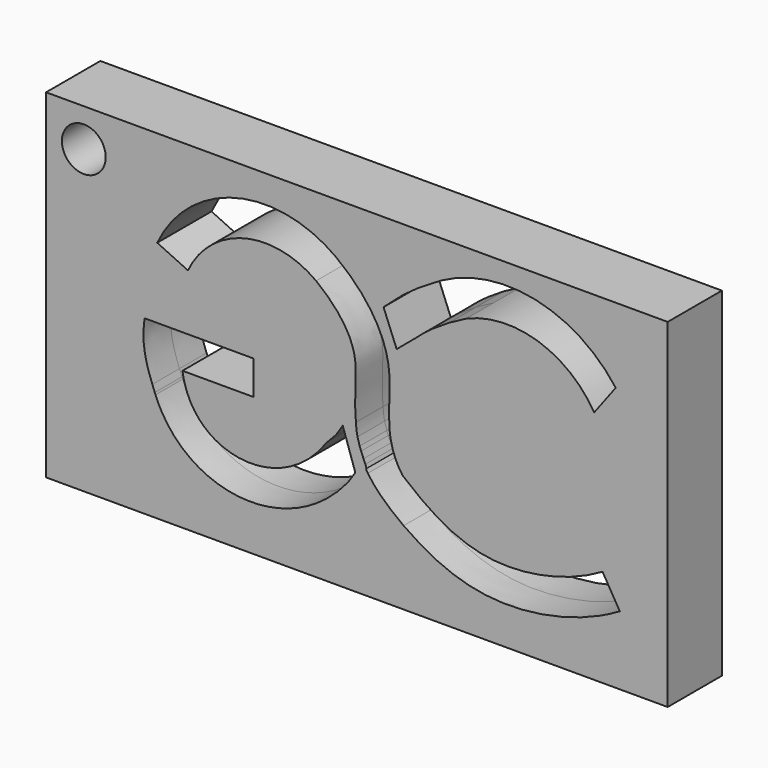
from build123d import *

# Parameters (mm, degrees)
F0_W     = 55
F0_H     = 30
F0_R     = 1.9388659874
F1_DEPTH = 3


# Not quite as in the source:
# - ends of sketch curves that miss each other by under 0.0002 mm in the source are joined
# - the dataset's text gives a spline's control points without its knots; the knots are read off the source's solid


with BuildPart() as f1:
    # F0 (on Front) → F1 (new body, symmetric)
    with BuildSketch(Plane.XZ):
        Rectangle(F0_W, F0_H)
        with Locations((-24.1624657065, 11.6540621966)):
            Circle(F0_R, mode=Mode.SUBTRACT)
        with BuildLine():
            ThreePointArc((-17.6640928467, 6.4768509395), (-10.685556205, 12.2426405249), (-1.8066326116, 10.4793994675))
            add(Edge.make_bspline(
                [(-1.8066326116, 10.4793994675), (0.9111458785, 8.4068691358), (4.1202484659, 3.5315186205), (2.1705021087, -1.9989735062), (4.045421263, -4.5930928496)],
                knots=[0, 0, 0, 0, 0.5094502434, 1, 1, 1, 1], degree=3))
            add(Edge.make_bspline(
                [(4.045421263, -4.5930928496), (6.4784704527, -6.6385440032), (11.4225557915, -9.8002947462), (18.8378328842, -8.054314346), (21.7365036724, -6.3367947143)],
                knots=[0, 0, 0, 0, 0.4804113206, 1, 1, 1, 1], degree=3))
            Line((21.7365036724, -6.3367947143), (23.2657495656, -8.9177648804))
            add(Edge.make_bspline(
                [(4.1382202245, -8.4692971196), (4.1624678344, -8.4865837301), (4.9099788848, -9.0175085674), (6.0687236287, -9.7483352983), (7.7170833942, -10.5320442339), (9.0266705688, -11.015570061), (10.1790279052, -11.3156937619), (11.1349042612, -11.4860935206), (12.1118572673, -11.6074297366), (13.3407082821, -11.6664441259), (15.3172141164, -11.5856834284), (17.7803139056, -11.1846498348), (20.641174588, -10.2819941321), (22.4229996015, -9.4171091932), (23.2657495656, -8.9177648804)],
                knots=[0.1208031529, 0.1208031529, 0.1208031529, 0.1208031529, 0.125, 0.25, 0.3125, 0.375, 0.4375, 0.46875, 0.5, 0.5625, 0.625, 0.75, 0.875, 0.9999989076, 0.9999989076, 0.9999989076, 0.9999989076], degree=3))
            add(Edge.make_bspline(
                [(0.9708350698, -5.4183705026), (1.6910337242, -6.5228260499), (2.8786849452, -7.5505327146), (4.1382202245, -8.4692971196)],
                knots=[0.5007210761, 0.5007210761, 0.5007210761, 0.5007210761, 1, 1, 1, 1], degree=3))
            add(Edge.make_bspline(
                [(0.7749087459, -5.0950080167), (0.8355835769, -5.2034973247), (0.9010125029, -5.3112945995), (0.9708350698, -5.4183705026)],
                knots=[0.4523164645, 0.4523164645, 0.4523164645, 0.4523164645, 0.5007210761, 0.5007210761, 0.5007210761, 0.5007210761], degree=3))
            add(Edge.make_bspline(
                [(0.6601995359, -4.87802362), (0.696432638, -4.9506366895), (0.7346227712, -5.0229748944), (0.7749087459, -5.0950080167)],
                knots=[0.4201774883, 0.4201774883, 0.4201774883, 0.4201774883, 0.4523164645, 0.4523164645, 0.4523164645, 0.4523164645], degree=3))
            add(Edge.make_bspline(
                [(0.6601995359, -4.87802362), (0.5457553685, -4.9921466011), (-0.197418957, -5.679000658), (-0.8276000802, -7.3815559883), (-3.5383820349, -9.5528269631), (-6.4036037178, -10.878806976), (-9.5175268759, -11.3250409398), (-12.5958587504, -10.8244366378), (-14.9118581064, -9.5196831868), (-16.4503468255, -7.9236394551), (-17.3737530763, -6.5629717915), (-17.9697890031, -5.3603946032), (-18.0825537585, -4.7711814756), (-18.0964615136, -4.6896541748)],
                knots=[0.0363625791, 0.0363625791, 0.0363625791, 0.0363625791, 0.0512646152, 0.1224303682, 0.2066568702, 0.2887928045, 0.3697104631, 0.4503939374, 0.5250439069, 0.5926719237, 0.6520324546, 0.7122837255, 0.7221646459, 0.7221646459, 0.7221646459, 0.7221646459], degree=3))
            add(Edge.make_bspline(
                [(-18.786193803, 0.233763308), (-19.1042212428, -1.8131556769), (-18.6276745861, -3.2945041185), (-18.0964615136, -4.6896541748)],
                knots=[0, 0, 0, 0, 4.8787183272, 4.8787183272, 4.8787183272, 4.8787183272], degree=3))
            Line((-18.786193803, 0.233763308), (-9.1412619867, 0.233763308))
            Line((-9.1412619867, 0.233763308), (-9.1412619867, -2.766236692))
            Line((-9.1412619867, -2.766236692), (-11.708700146, -2.766236692))
            add(Edge.make_bspline(
                [(-11.708700146, -2.766236692), (-8.4560263125, -2.815236385), (-4.719044159, -3.0335808655), (-2.1487066373, -3.3793081037)],
                knots=[0.87686085, 0.87686085, 0.87686085, 0.87686085, 0.9540771145, 0.9540771145, 0.9540771145, 0.9540771145], degree=3))
            add(Edge.make_bspline(
                [(-2.1487066373, -3.3793081037), (-2.0687729336, -3.3900597106), (-1.9899675131, -3.4009345117), (-1.9123400298, -3.4119312449)],
                knots=[0.9540771145, 0.9540771145, 0.9540771145, 0.9540771145, 0.9564784264, 0.9564784264, 0.9564784264, 0.9564784264], degree=3))
            Line((-1.9123400298, -3.4119312449), (-1.8364996879, -3.3321739989))
            Line((-1.8364996879, -3.3321739989), (-1.2497392903, -2.4288706426))
            Line((-1.2497392903, -2.4288706426), (-0.8619702149, -3.5822052172))
            add(Edge.make_bspline(
                [(-0.8619702149, -3.5822052172), (-0.4110593021, -3.6667089832), (-0.0287691917, -3.7568014187), (0.2682413254, -3.8520591098)],
                knots=[0.9682440451, 0.9682440451, 0.9682440451, 0.9682440451, 0.9849297687, 0.9849297687, 0.9849297687, 0.9849297687], degree=3))
            add(Edge.make_bspline(
                [(0.0566001038, -2.8747222202), (0.1099315572, -3.2013897212), (0.1766725727, -3.5279972379), (0.2682413254, -3.8520591098)],
                knots=[0.1312140251, 0.1312140251, 0.1312140251, 0.1312140251, 0.2709870602, 0.2709870602, 0.2709870602, 0.2709870602], degree=3))
            add(Edge.make_bspline(
                [(-0.0856948489, -1.7935240537), (-0.0651666036, -2.2040296052), (-0.0140771955, -2.5577803712), (0.0566001038, -2.8747222202)],
                knots=[0, 0, 0, 0, 0.9044663432, 0.9044663432, 0.9044663432, 0.9044663432], degree=3))
            add(Edge.make_bspline(
                [(-3.6107100667, 8.0823726543), (-3.0624362988, 7.6631509681), (-2.0964601547, 6.8016967531), (-1.2314902531, 5.7195620145), (-0.7330802188, 4.8707855584), (-0.4512938807, 4.2466244067), (-0.287727537, 3.7365048832), (-0.1965285589, 3.3315021794), (-0.1475436674, 3.0291795886), (-0.1171491383, 2.7232253787), (-0.1006872263, 2.367601974), (-0.098417222, 1.9711308495), (-0.1106132344, 1.3862202996), (-0.1452655215, 0.5543107318), (-0.1679299933, -0.5614993222), (-0.1282499701, -1.3843821047), (-0.0856948489, -1.7935240537)],
                knots=[0.0011339683, 0.0011339683, 0.0011339683, 0.0011339683, 0.125, 0.25, 0.3125, 0.375, 0.4375, 0.46875, 0.5, 0.53125, 0.5625, 0.59375, 0.625, 0.6875, 0.75, 0.8064342098, 0.8064342098, 0.8064342098, 0.8064342098], degree=3))
            ThreePointArc((-3.6107100667, 8.0823726543), (-9.9597048312, 9.3317569254), (-14.9458452328, 5.2075479372))
            Line((-14.9458452328, 5.2075479372), (-17.6640928467, 6.4768509395))
        make_face(mode=Mode.SUBTRACT)
        with BuildLine():
            ThreePointArc((7.44970433, 11.7041880822), (15.7997813856, 12.9273848123), (22.9030745256, 8.3707167705))
            Line((22.9030745256, 8.3707167705), (20.9994814153, 5.8342256079))
            ThreePointArc((20.9994814153, 5.8342256079), (16.0174548232, 9.7676245314), (9.6773733101, 9.4584603969))
            add(Edge.make_bspline(
                [(8.1585890684, 8.6435706468), (8.6642005474, 8.9163421832), (9.1717618311, 9.1856888605), (9.6773733101, 9.4584603969)],
                knots=[0, 0, 0, 0, 1.7235866319, 1.7235866319, 1.7235866319, 1.7235866319], degree=3))
            add(Edge.make_bspline(
                [(8.1585890684, 8.6435706468), (7.6831365183, 8.357623282), (6.9919675002, 7.9139890407), (6.2840136703, 7.4063154618), (5.8111423105, 7.0306922773), (5.4983866823, 6.7579836155), (5.3208850022, 6.5956781542), (5.2582055037, 6.5378467511)],
                knots=[0.0833975483, 0.0833975483, 0.0833975483, 0.0833975483, 0.25, 0.375, 0.5, 0.625, 0.692347247, 0.692347247, 0.692347247, 0.692347247], degree=3))
            add(Edge.make_bspline(
                [(5.2582055037, 6.5378467511), (4.6790308276, 6.0521310033), (4.099855095, 5.5664163998), (3.5206793628, 5.0807017966)],
                knots=[0, 0, 0, 0, 2.2676571264, 2.2676571264, 2.2676571264, 2.2676571264], degree=3))
            Line((3.5206793628, 5.0807017966), (2.3603189094, 7.9763170318))
            add(Edge.make_bspline(
                [(7.44970433, 11.7041880822), (3.8568143179, 9.6563175042), (3.3117315552, 8.7162573024), (2.3603189094, 7.9763170318)],
                knots=[0, 0, 0, 0, 6.3086342839, 6.3086342839, 6.3086342839, 6.3086342839], degree=3))
        make_face(mode=Mode.SUBTRACT)
        with BuildLine():
            add(Edge.make_bspline(
                [(0.0566001038, -2.8747222202), (0.1099973475, -3.1141742265), (0.1745752004, -3.332616002), (0.2456015748, -3.5386489562)],
                knots=[0.9044663432, 0.9044663432, 0.9044663432, 0.9044663432, 1.5877976268, 1.5877976268, 1.5877976268, 1.5877976268], degree=3))
            add(Edge.make_bspline(
                [(0.0566001038, -2.8747222202), (0.1099315572, -3.2013897212), (0.1766725727, -3.5279972379), (0.2682413254, -3.8520591098)],
                knots=[0.1312140251, 0.1312140251, 0.1312140251, 0.1312140251, 0.2709870602, 0.2709870602, 0.2709870602, 0.2709870602], degree=3))
            add(Edge.make_bspline(
                [(0.2682413254, -3.8520591098), (0.2963348926, -3.8610693239), (0.3236654761, -3.8701257507), (0.3502189783, -3.879228032)],
                knots=[0.9849297687, 0.9849297687, 0.9849297687, 0.9849297687, 0.9865080344, 0.9865080344, 0.9865080344, 0.9865080344], degree=3))
            add(Edge.make_bspline(
                [(0.2456015748, -3.5386489562), (0.2779370037, -3.6516481268), (0.3127699679, -3.7652394685), (0.3502189794, -3.8792280306)],
                knots=[0.8826192036, 0.8826192036, 0.8826192036, 0.8826192036, 0.8968376779, 0.8968376779, 0.8968376779, 0.8968376779], degree=3))
        make_face()
        with BuildLine():
            add(Edge.make_bspline(
                [(0.2456015748, -3.5386489562), (0.2869994632, -3.6587357455), (0.3305880231, -3.7746070492), (0.3754302784, -3.8879659872)],
                knots=[1.5877976268, 1.5877976268, 1.5877976268, 1.5877976268, 1.9860788639, 1.9860788639, 1.9860788639, 1.9860788639], degree=3))
            add(Edge.make_bspline(
                [(0.2456015748, -3.5386489562), (0.2779370037, -3.6516481268), (0.3127699679, -3.7652394685), (0.3502189794, -3.8792280306)],
                knots=[0.8826192036, 0.8826192036, 0.8826192036, 0.8826192036, 0.8968376779, 0.8968376779, 0.8968376779, 0.8968376779], degree=3))
            add(Edge.make_bspline(
                [(0.3502189783, -3.879228032), (0.3587022152, -3.8821360028), (0.3671061389, -3.8850486538), (0.3754302895, -3.8879659732)],
                knots=[0.9865080344, 0.9865080344, 0.9865080344, 0.9865080344, 0.9870122542, 0.9870122542, 0.9870122542, 0.9870122542], degree=3))
        make_face()
        with BuildLine():
            add(Edge.make_bspline(
                [(0.2682413254, -3.8520591098), (0.3659796439, -4.1979550785), (0.49200401, -4.540950814), (0.6601995359, -4.87802362)],
                knots=[0.2709870602, 0.2709870602, 0.2709870602, 0.2709870602, 0.4201774883, 0.4201774883, 0.4201774883, 0.4201774883], degree=3))
            add(Edge.make_bspline(
                [(-0.8619702149, -3.5822052172), (-0.4110593021, -3.6667089832), (-0.0287691917, -3.7568014187), (0.2682413254, -3.8520591098)],
                knots=[0.9682440451, 0.9682440451, 0.9682440451, 0.9682440451, 0.9849297687, 0.9849297687, 0.9849297687, 0.9849297687], degree=3))
            Line((-0.8619702149, -3.5822052172), (-0.1403129716, -5.7286173534))
            Line((-0.1403129716, -5.7286173534), (-0.8010316837, -6.7117390489))
            add(Edge.make_bspline(
                [(-0.8010316837, -6.7117390489), (-0.9057419923, -6.8407558065), (-1.7555380998, -7.8476748795), (-3.5696809972, -9.4107976412), (-6.4669061446, -10.7392262424), (-9.5308170044, -11.1654358176), (-12.5637321995, -10.6552078651), (-14.8767946166, -9.3977719697), (-16.416248249, -7.8815514015), (-17.2610915999, -6.6532656573), (-17.6698693055, -5.7874242382), (-17.8146100334, -5.4216091132)],
                knots=[0.1070652908, 0.1070652908, 0.1070652908, 0.1070652908, 0.125, 0.25, 0.375, 0.5, 0.625, 0.75, 0.8125, 0.875, 0.9179074804, 0.9179074804, 0.9179074804, 0.9179074804], degree=3))
            add(Edge.make_bspline(
                [(-17.8146100334, -5.4216091132), (-17.836650687, -5.3659039596), (-17.858189141, -5.3098889382), (-17.8792200637, -5.2535723059)],
                knots=[0.9179074804, 0.9179074804, 0.9179074804, 0.9179074804, 0.9244412939, 0.9244412939, 0.9244412939, 0.9244412939], degree=3))
            add(Edge.make_bspline(
                [(-18.0964615131, -4.6896541747), (-18.0244379036, -4.878813192), (-17.9514093709, -5.0663876394), (-17.8792200637, -5.2535723059)],
                knots=[4.8787183272, 4.8787183272, 4.8787183272, 4.8787183272, 5.5401909482, 5.5401909482, 5.5401909482, 5.5401909482], degree=3))
            add(Edge.make_bspline(
                [(0.6601995359, -4.87802362), (0.5457553685, -4.9921466011), (-0.197418957, -5.679000658), (-0.8276000802, -7.3815559883), (-3.5383820349, -9.5528269631), (-6.4036037178, -10.878806976), (-9.5175268759, -11.3250409398), (-12.5958587504, -10.8244366378), (-14.9118581064, -9.5196831868), (-16.4503468255, -7.9236394551), (-17.3737530763, -6.5629717915), (-17.9697890031, -5.3603946032), (-18.0825537585, -4.7711814756), (-18.0964615131, -4.6896541747)],
                knots=[0.0363625791, 0.0363625791, 0.0363625791, 0.0363625791, 0.0512646152, 0.1224303682, 0.2066568702, 0.2887928045, 0.3697104631, 0.4503939374, 0.5250439069, 0.5926719237, 0.6520324546, 0.7122837255, 0.7221646459, 0.7221646459, 0.7221646459, 0.7221646459], degree=3))
        make_face()
        with BuildLine():
            add(Edge.make_bspline(
                [(0.2682413254, -3.8520591098), (0.2963348926, -3.8610693239), (0.3236654761, -3.8701257507), (0.3502189783, -3.879228032)],
                knots=[0.9849297687, 0.9849297687, 0.9849297687, 0.9849297687, 0.9865080344, 0.9865080344, 0.9865080344, 0.9865080344], degree=3))
            add(Edge.make_bspline(
                [(0.2682413254, -3.8520591098), (0.3659796439, -4.1979550785), (0.49200401, -4.540950814), (0.6601995359, -4.87802362)],
                knots=[0.2709870602, 0.2709870602, 0.2709870602, 0.2709870602, 0.4201774883, 0.4201774883, 0.4201774883, 0.4201774883], degree=3))
            add(Edge.make_bspline(
                [(0.6960921253, -4.8418824987), (0.6843093612, -4.8538758822), (0.6723344504, -4.8659227621), (0.6601995359, -4.87802362)],
                knots=[0.0347824642, 0.0347824642, 0.0347824642, 0.0347824642, 0.0363625791, 0.0363625791, 0.0363625791, 0.0363625791], degree=3))
            add(Edge.make_bspline(
                [(0.6245644861, -4.5631799108), (0.6469595886, -4.6596538389), (0.6707650709, -4.7524516706), (0.6960921437, -4.8418825074)],
                knots=[0.3698951151, 0.3698951151, 0.3698951151, 0.3698951151, 0.6175600106, 0.6175600106, 0.6175600106, 0.6175600106], degree=3))
            add(Edge.make_bspline(
                [(0.5893817819, -4.4030555634), (0.600706987, -4.45754263), (0.6124286562, -4.5109010168), (0.6245644861, -4.5631799108)],
                knots=[0.2356863492, 0.2356863492, 0.2356863492, 0.2356863492, 0.3698951151, 0.3698951151, 0.3698951151, 0.3698951151], degree=3))
            add(Edge.make_bspline(
                [(0.3754302784, -3.8879659872), (0.4448998148, -4.0635814378), (0.5173782388, -4.233167174), (0.5893817819, -4.4030555634)],
                knots=[1.9860788639, 1.9860788639, 1.9860788639, 1.9860788639, 2.6030953967, 2.6030953967, 2.6030953967, 2.6030953967], degree=3))
            add(Edge.make_bspline(
                [(0.3502189783, -3.879228032), (0.3587022152, -3.8821360028), (0.3671061389, -3.8850486538), (0.3754302895, -3.8879659732)],
                knots=[0.9865080344, 0.9865080344, 0.9865080344, 0.9865080344, 0.9870122542, 0.9870122542, 0.9870122542, 0.9870122542], degree=3))
        make_face()
        with BuildLine():
            add(Edge.make_bspline(
                [(0.6601995359, -4.87802362), (0.696432638, -4.9506366895), (0.7346227712, -5.0229748944), (0.7749087459, -5.0950080167)],
                knots=[0.4201774883, 0.4201774883, 0.4201774883, 0.4201774883, 0.4523164645, 0.4523164645, 0.4523164645, 0.4523164645], degree=3))
            add(Edge.make_bspline(
                [(0.6960921437, -4.8418825074), (0.720872959, -4.929384489), (0.7471104369, -5.013663149), (0.7749087459, -5.0950080167)],
                knots=[0.6175600106, 0.6175600106, 0.6175600106, 0.6175600106, 0.8598832396, 0.8598832396, 0.8598832396, 0.8598832396], degree=3))
            add(Edge.make_bspline(
                [(0.6960921253, -4.8418824987), (0.6843093612, -4.8538758822), (0.6723344504, -4.8659227621), (0.6601995359, -4.87802362)],
                knots=[0.0347824642, 0.0347824642, 0.0347824642, 0.0347824642, 0.0363625791, 0.0363625791, 0.0363625791, 0.0363625791], degree=3))
        make_face()
        with BuildLine():
            add(Edge.make_bspline(
                [(0.6960921437, -4.8418825074), (0.720872959, -4.929384489), (0.7471104369, -5.013663149), (0.7749087459, -5.0950080167)],
                knots=[0.6175600106, 0.6175600106, 0.6175600106, 0.6175600106, 0.8598832396, 0.8598832396, 0.8598832396, 0.8598832396], degree=3))
            Line((0.7749087459, -5.0950080167), (0.8604262998, -5.0818839093))
            add(Edge.make_bspline(
                [(0.7486387865, -4.7872831293), (0.7870430822, -4.8835798968), (0.8245028318, -4.9814216287), (0.8604262998, -5.0818839093)],
                knots=[3.0644343463, 3.0644343463, 3.0644343463, 3.0644343463, 3.4061432185, 3.4061432185, 3.4061432185, 3.4061432185], degree=3))
            add(Edge.make_bspline(
                [(0.7486387865, -4.7872831293), (0.7316481919, -4.8053591866), (0.7140944253, -4.8235584037), (0.6960921253, -4.8418824987)],
                knots=[0.0323682852, 0.0323682852, 0.0323682852, 0.0323682852, 0.0347824642, 0.0347824642, 0.0347824642, 0.0347824642], degree=3))
        make_face()
        with BuildLine():
            add(Edge.make_bspline(
                [(0.6245644861, -4.5631799108), (0.6469595886, -4.6596538389), (0.6707650709, -4.7524516706), (0.6960921437, -4.8418825074)],
                knots=[0.3698951151, 0.3698951151, 0.3698951151, 0.3698951151, 0.6175600106, 0.6175600106, 0.6175600106, 0.6175600106], degree=3))
            add(Edge.make_bspline(
                [(0.7486387865, -4.7872831293), (0.7316481919, -4.8053591866), (0.7140944253, -4.8235584037), (0.6960921253, -4.8418824987)],
                knots=[0.0323682852, 0.0323682852, 0.0323682852, 0.0323682852, 0.0347824642, 0.0347824642, 0.0347824642, 0.0347824642], degree=3))
            add(Edge.make_bspline(
                [(0.5893817819, -4.4030555634), (0.6432183278, -4.5300799249), (0.6967893941, -4.6572734832), (0.7486387865, -4.7872831293)],
                knots=[2.6030953967, 2.6030953967, 2.6030953967, 2.6030953967, 3.0644343463, 3.0644343463, 3.0644343463, 3.0644343463], degree=3))
            add(Edge.make_bspline(
                [(0.5893817819, -4.4030555634), (0.600706987, -4.45754263), (0.6124286562, -4.5109010168), (0.6245644861, -4.5631799108)],
                knots=[0.2356863492, 0.2356863492, 0.2356863492, 0.2356863492, 0.3698951151, 0.3698951151, 0.3698951151, 0.3698951151], degree=3))
        make_face()
        with BuildLine():
            Line((-2.6718280506, -4.2106443235), (-1.9123400298, -3.411931245))
            add(Edge.make_bspline(
                [(-2.1487066373, -3.3793081037), (-2.0687729336, -3.3900597106), (-1.9899675131, -3.4009345117), (-1.9123400298, -3.4119312449)],
                knots=[0.9540771145, 0.9540771145, 0.9540771145, 0.9540771145, 0.9564784264, 0.9564784264, 0.9564784264, 0.9564784264], degree=3))
            add(Edge.make_bspline(
                [(-2.1487066341, -3.3793081236), (-2.3142498584, -3.6703682853), (-2.4889581982, -3.9474567137), (-2.6718280506, -4.2106443235)],
                knots=[0.0284049411, 0.0284049411, 0.0284049411, 0.0284049411, 0.0719169232, 0.0719169232, 0.0719169232, 0.0719169232], degree=3))
        make_face()
        with BuildLine():
            add(Edge.make_bspline(
                [(-2.1487066341, -3.3793081236), (-2.3142498584, -3.6703682853), (-2.4889581982, -3.9474567137), (-2.6718280506, -4.2106443235)],
                knots=[0.0284049411, 0.0284049411, 0.0284049411, 0.0284049411, 0.0719169232, 0.0719169232, 0.0719169232, 0.0719169232], degree=3))
            add(Edge.make_bspline(
                [(-11.708700146, -2.766236692), (-8.4560263125, -2.815236385), (-4.719044159, -3.0335808655), (-2.1487066373, -3.3793081037)],
                knots=[0.87686085, 0.87686085, 0.87686085, 0.87686085, 0.9540771145, 0.9540771145, 0.9540771145, 0.9540771145], degree=3))
            Line((-11.708700146, -2.766236692), (-14.3142643113, -2.766236692))
            add(Edge.make_bspline(
                [(-15.4257163185, -2.7971153139), (-15.0758805399, -2.7833546677), (-14.7039846687, -2.773097679), (-14.3142643113, -2.766236692)],
                knots=[0.8444576318, 0.8444576318, 0.8444576318, 0.8444576318, 0.8550282995, 0.8550282995, 0.8550282995, 0.8550282995], degree=3))
            add(Edge.make_bspline(
                [(-2.6718280506, -4.2106443235), (-4.6042931453, -6.9918620195), (-10.3350499454, -9.4682617557), (-14.9575381248, -5.9809362104), (-15.4257163186, -2.7971153145)],
                knots=[0.0719169232, 0.0719169232, 0.0719169232, 0.0719169232, 0.5317269228, 0.9984931862, 0.9984931862, 0.9984931862, 0.9984931862], degree=3))
        make_face()
        with BuildLine():
            add(Edge.make_bspline(
                [(-15.4257163186, -2.7971153145), (-15.4272276903, -2.7868373112), (-15.4287196742, -2.7765444361), (-15.4301922171, -2.766236692)],
                knots=[0.9984931862, 0.9984931862, 0.9984931862, 0.9984931862, 1, 1, 1, 1], degree=3))
            add(Edge.make_bspline(
                [(-15.4257163185, -2.7971153139), (-15.0758805399, -2.7833546677), (-14.7039846687, -2.773097679), (-14.3142643113, -2.766236692)],
                knots=[0.8444576318, 0.8444576318, 0.8444576318, 0.8444576318, 0.8550282995, 0.8550282995, 0.8550282995, 0.8550282995], degree=3))
            Line((-14.3142643113, -2.766236692), (-15.4301922171, -2.766236692))
        make_face()
    extrude(amount=F1_DEPTH, both=True)


solid = f1.part
